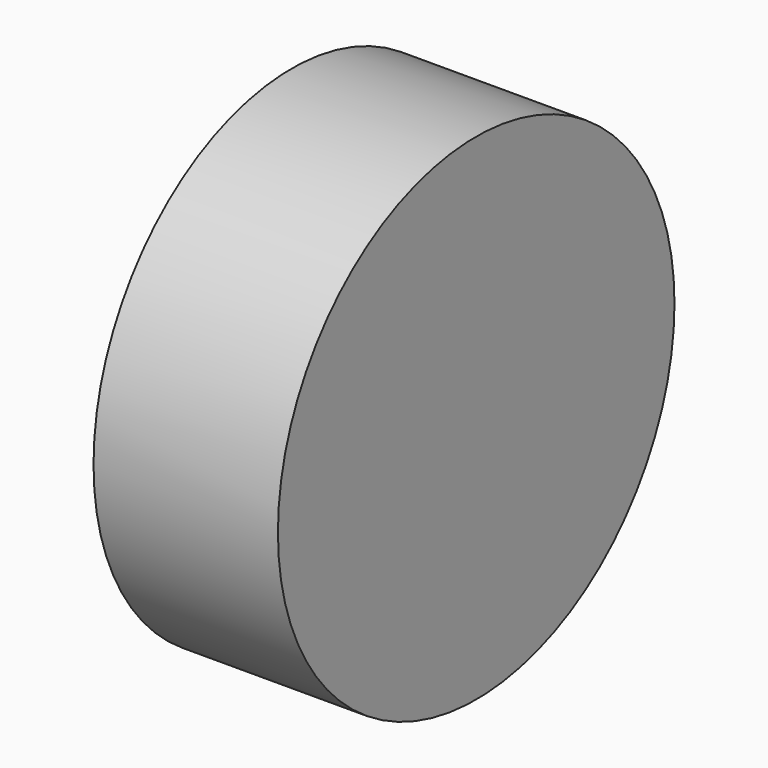
from build123d import *

# Parameters (mm, degrees)
F0_R     = 121.9740608537
F1_DEPTH = 90.7566379756


# Not quite as in the source:
# - the program builds the solid bodies; features that only make, move or delete a surface that nothing else refers to are left out


with BuildPart() as f1:
    # F0 (on Right) → F1 (new body)
    with BuildSketch(Plane.YZ):
        with Locations((0, 88.6222869158)):
            Circle(F0_R)
    extrude(amount=F1_DEPTH)


solid = f1.part
